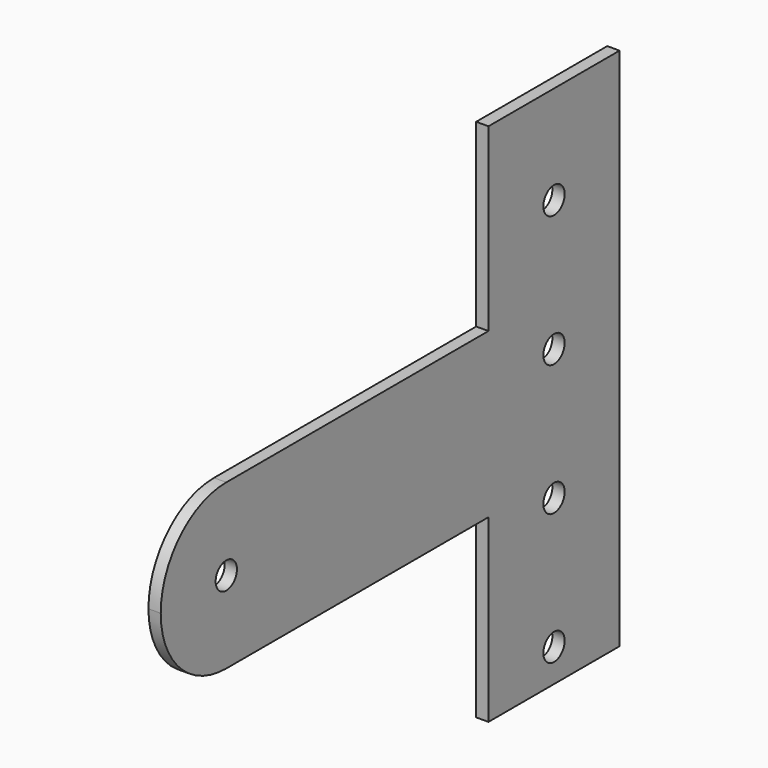
from build123d import *

# Parameters (mm, degrees)
F0_W     = 127
F0_H     = 406.4
F1_DEPTH = 9.525
F3_DEPTH = 9.525
F4_R     = 63.49999
F6_D     = 20.6375
F8_D     = 20.6375


# Not quite as in the source:
# - a fillet or chamfer is up to 0.001 mm smaller than in the source, because OpenCascade refuses the exact size
# - a length typed as a fraction of an inch, garbled in the dataset ("3 / 203.2 mm" for 3/8 in), is restored


with BuildPart() as f1:
    # F0 (on Right) → F1 (new body)
    with BuildSketch(Plane.YZ):
        with Locations((26.2075642347, 169.2136289895)):
            Rectangle(F0_W, F0_H)
    extrude(amount=F1_DEPTH)

    # F2 (on face) → F3 (join)
    with BuildSketch(Plane.YZ.offset(9.525)):
        Polygon((-37.2924357653, 105.7136289895), (-37.2924357653, 169.2136289895), (-37.2924357653, 232.7136289895), (-354.7924357653, 232.7136289895), (-354.7924357653, 105.7136289895), align=None)
    extrude(amount=-F3_DEPTH)

    # F4 (radius 63.5 in the source; OpenCascade refuses exactly that, so slightly less here)
    f4_edges = [f1.edges().sort_by_distance(p)[0] for p in [
        (4.7625, -354.792436, 232.713629),
        (4.7625, -354.792436, 105.713629),
    ]]
    fillet(f4_edges, radius=F4_R)

    # F6 (through all)
    with Locations(Plane.YZ.offset(9.525)):
        with Locations((-291.2924357653, 169.2136289895)):
            Hole(F6_D / 2)

    # F8 (through all)
    with Locations(Plane.YZ.offset(9.525)):
        with Locations((26.2075642347, 296.2136289895), (26.2075642347, 194.6136289895), (26.2075642347, 93.0136289895), (26.2075642347, -8.5863710105)):
            Hole(F8_D / 2)


solid = f1.part
